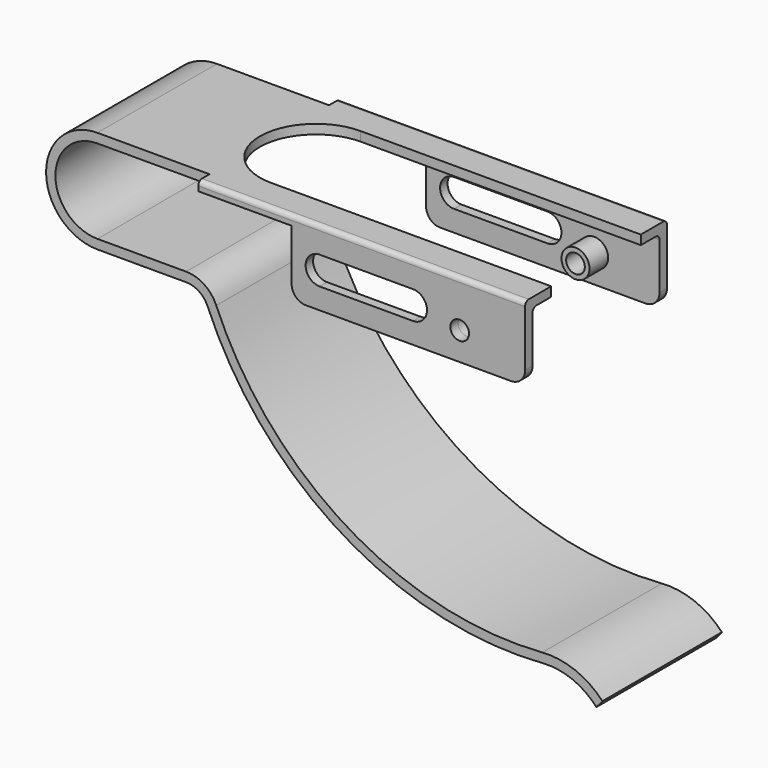
from build123d import *

# Parameters (mm, degrees)
F1_DEPTH  = 16
F2_W      = 70
F2_H      = 3
F3_DEPTH  = 2
F4_W      = 50
F4_H      = 14
F5_DEPTH  = 2
F6_R      = 1
F9_DEPTH  = 4
F11_DEPTH = 38.001
F13_D     = 4
F14_R     = 3
F14_R_2   = 2
F15_DEPTH = 5
F16_R     = 3


# Not quite as in the source:
# - a pattern or mirror of a feature is missing from the dataset's text; its kind, count and spacing are read off the source's solid


with BuildPart() as f1:
    # F0 (on Front) → F1 (new body)
    with BuildSketch(Plane.XZ):
        with BuildLine():
            Line((94, 11), (0, 11))
            ThreePointArc((0, 11), (-11, 0), (0, -11))
            Line((0, -11), (19, -11))
            ThreePointArc((19, -11), (21.7681124643, -11.8361612201), (23.6103896104, -14.064978646))
            ThreePointArc((23.6103896104, -14.064978646), (52.4378053116, -47.6260855158), (95.4479042723, -57.9942665386))
            ThreePointArc((95.4479042723, -57.9942665386), (101.6870615127, -58.9476250352), (106.8734428361, -62.5444881493))
            Line((106.8734428361, -62.5444881493), (108.1694222725, -61))
            ThreePointArc((108.1694222725, -61), (102.3002117906, -57.039668375), (95.2965735981, -56))
            ThreePointArc((95.2965735981, -56), (53.4811996085, -45.9198240056), (25.4545454545, -13.2909701044))
            ThreePointArc((25.4545454545, -13.2909701044), (22.87535745, -10.1706257081), (19, -9))
            Line((19, -9), (0, -9))
            ThreePointArc((0, -9), (-9, 0), (0, 9))
            Line((0, 9), (94, 9))
            Line((94, 9), (94, 11))
        make_face()
    extrude(amount=F1_DEPTH)

    # F2 (on face) → F3 (join)
    with BuildSketch(Plane.XY.offset(11)):
        with Locations((59, -17.5)):
            Rectangle(F2_W, F2_H)
    extrude(amount=-F3_DEPTH)

    # F4 (on face) → F5 (join)
    with BuildSketch(Plane.XZ.offset(19)):
        with Locations((69, 2)):
            Rectangle(F4_W, F4_H)
    extrude(amount=-F5_DEPTH)

    # F6
    f6_edges = [f1.edges().sort_by_distance(p)[0] for p in [
        (59, -19, 11),
        (69, -17, 9),
    ]]
    fillet(f6_edges, radius=F6_R)

    # F7: F1 across plane


with BuildPart() as f1_1:
    add(f1.part)
    add(f1.part.mirror(Plane.XZ))

    # F8 (on face) → F9 (cut)
    with BuildSketch(Plane.XY.offset(11)):
        with BuildLine():
            Line((94, 12), (34, 12))
            ThreePointArc((34, 12), (22, 0), (34, -12))
            Line((34, -12), (94, -12))
            Line((94, -12), (94, 12))
        make_face()
    extrude(amount=-F9_DEPTH, mode=Mode.SUBTRACT)

    # F10 (on face) → F11 (cut, through all)
    with BuildSketch(Plane.XZ.offset(19)):
        with BuildLine():
            ThreePointArc((70, -0.5), (73, 2.5), (70, 5.5))
            Line((70, 5.5), (50, 5.5))
            ThreePointArc((50, 5.5), (47, 2.5), (50, -0.5))
            Line((50, -0.5), (70, -0.5))
        make_face()
    extrude(amount=-F11_DEPTH, mode=Mode.SUBTRACT)

    # F13 (through all)
    with Locations(Plane.XZ.offset(19)):
        with Locations((80, 1)):
            Hole(F13_D / 2)

    # F14 (on face) → F15 (join)
    with BuildSketch(Plane(origin=(0, -17, 0), x_dir=(-1, 0, 0), z_dir=(0, 1, 0))):
        with Locations((-80, 1)):
            Circle(F14_R)
        with Locations((-80, 1)):
            Circle(F14_R_2, mode=Mode.SUBTRACT)
    f15 = extrude(amount=F15_DEPTH)

    # F15_copies: F15 across plane
    add(f15.mirror(Plane.ZX))

    # F16
    f16_edges = [f1_1.edges().sort_by_distance(p)[0] for p in [
        (94, 18, -5),
        (44, 18, -5),
        (94, -18, -5),
        (44, -18, -5),
    ]]
    fillet(f16_edges, radius=F16_R)


solid = f1_1.part
